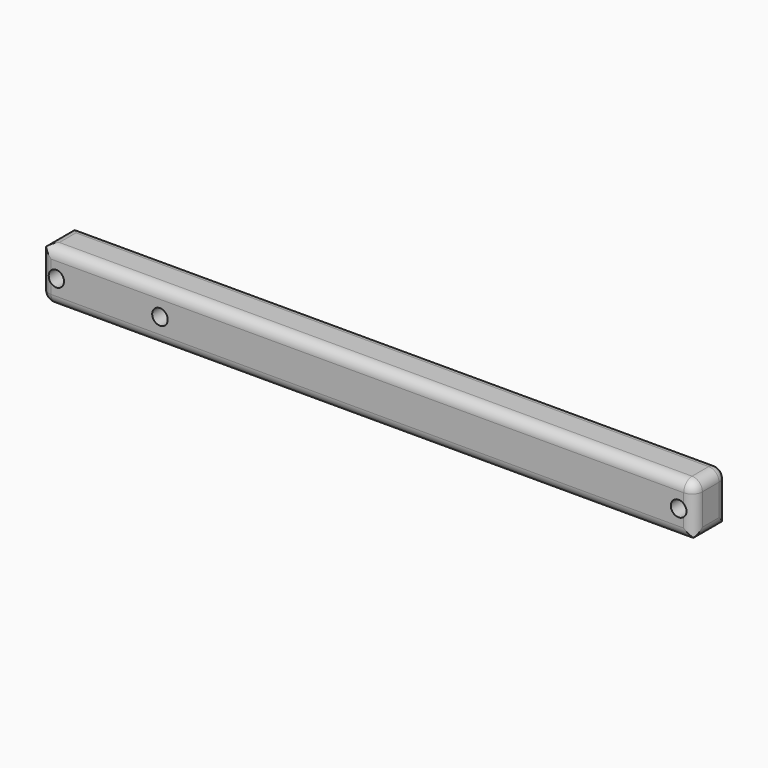
from build123d import *

# Parameters (mm, degrees)
F0_W         = 126
F0_H         = 10
F0_R         = 1.5
F1_DEPTH     = 8
F2_T1_DEPTH  = 4
F2_T3_DEPTH  = 18
F2_T5_DEPTH  = 129
F2_T7_DEPTH  = 13
F2_S11_W     = 2
F2_S11_H     = 2
F2_T12_DEPTH = 2
F2_S17_W     = 2
F2_S17_H     = 2
F2_T18_DEPTH = 2
F3_T1_DEPTH  = 11
F3_T3_DEPTH  = 4
F3_T5_DEPTH  = 127
F3_S9_W      = 2.04
F3_S9_H      = 2.04
F3_T10_DEPTH = 2.04
F3_S15_W     = 2.04
F3_S15_H     = 2.04
F3_T16_DEPTH = 2.04


# Not quite as in the source:
# - a fillet or chamfer that OpenCascade refuses, or shapes differently, is made with other operations: its cross-section is extruded or revolved along the edge and cut away or added


with BuildPart() as f1:
    # F0 (on Front) → F1 (new body)
    with BuildSketch(Plane.XZ):
        with Locations((0, 5)):
            Rectangle(F0_W, F0_H)
        with Locations((-60, 5)):
            Circle(F0_R, mode=Mode.SUBTRACT)
        with Locations((-40, 5)):
            Circle(F0_R, mode=Mode.SUBTRACT)
        with Locations((60, 5)):
            Circle(F0_R, mode=Mode.SUBTRACT)
    extrude(amount=F1_DEPTH)

    # F2: fillet of radius 2 on 7 edges, made by hand

    # F2_s2 → F2_t1 (cut)
    with BuildSketch(Plane.XZ.offset(2)):
        with BuildLine():
            ThreePointArc((63, 8), (62.4142135624, 9.4142135624), (61, 10))
            Line((61, 10), (63, 10))
            Line((63, 10), (63, 8))
        make_face()
    extrude(amount=F2_T1_DEPTH, mode=Mode.SUBTRACT)

    # F2_s4 → F2_t3 (cut)
    with BuildSketch(Plane.XZ.offset(-5)):
        with BuildLine():
            ThreePointArc((-63, 8), (-62.4142135624, 9.4142135624), (-61, 10))
            Line((-61, 10), (-63, 10))
            Line((-63, 10), (-63, 8))
        make_face()
        with BuildLine():
            ThreePointArc((61, 0), (62.4142135624, 0.5857864376), (63, 2))
            Line((63, 2), (63, 0))
            Line((63, 0), (61, 0))
        make_face()
    extrude(amount=F2_T3_DEPTH, mode=Mode.SUBTRACT)

    # F2_s6 → F2_t5 (cut)
    with BuildSketch(Plane.YZ.offset(-68)):
        with BuildLine():
            ThreePointArc((-2, 10), (-0.5857864376, 9.4142135624), (0, 8))
            Line((0, 8), (0, 10))
            Line((0, 10), (-2, 10))
        make_face()
        with BuildLine():
            ThreePointArc((-6, 10), (-7.4142135624, 9.4142135624), (-8, 8))
            Line((-8, 8), (-8, 10))
            Line((-8, 10), (-6, 10))
        make_face()
    extrude(amount=F2_T5_DEPTH, mode=Mode.SUBTRACT)

    # F2_s8 → F2_t7 (cut)
    with BuildSketch(Plane.XY.offset(-5)):
        with BuildLine():
            ThreePointArc((63, -2), (62.4142135624, -0.5857864376), (61, 0))
            Line((61, 0), (63, 0))
            Line((63, 0), (63, -2))
        make_face()
        with BuildLine():
            ThreePointArc((63, -6), (62.4142135624, -7.4142135624), (61, -8))
            Line((61, -8), (63, -8))
            Line((63, -8), (63, -6))
        make_face()
    extrude(amount=F2_T7_DEPTH, mode=Mode.SUBTRACT)


with BuildPart() as f2_tool10:
    # F2_s11 → F2_t12 (new body)
    with BuildSketch(Plane.YZ.offset(61)):
        with Locations((-1, 9)):
            Rectangle(F2_S11_W, F2_S11_H)
    extrude(amount=F2_T12_DEPTH)

    # F2_s13 → F2_t14 (revolve, cut)
    with BuildSketch(Plane(origin=(61, -2, 8), x_dir=(0, -0.7071067812, -0.7071067812), z_dir=(0, -0.7071067812, 0.7071067812))):
        with BuildLine():
            ThreePointArc((0, -2), (2, 0), (0, 2))
            Line((0, 2), (0, -2))
        make_face()
    revolve(axis=Axis((61, -2, 8), (1, 0, 0)), mode=Mode.SUBTRACT)


with BuildPart() as f1_1:
    add(f1.part)

    # F2_t9: cut F2_tool10
    add(f2_tool10.part, mode=Mode.SUBTRACT)


with BuildPart() as f2_tool16:
    # F2_s17 → F2_t18 (new body)
    with BuildSketch(Plane.XZ.offset(6)):
        with Locations((62, 9)):
            Rectangle(F2_S17_W, F2_S17_H)
    extrude(amount=F2_T18_DEPTH)

    # F2_s19 → F2_t20 (revolve, cut)
    with BuildSketch(Plane(origin=(61, -6, 8), x_dir=(-0.7071067812, 0, -0.7071067812), z_dir=(-0.7071067812, 0, 0.7071067812))):
        with BuildLine():
            ThreePointArc((0, -2), (2, 0), (0, 2))
            Line((0, 2), (0, -2))
        make_face()
    revolve(axis=Axis((61, -6, 8), (0, -1, 0)), mode=Mode.SUBTRACT)


with BuildPart() as f1_2:
    add(f1_1.part)

    # F2_t15: cut F2_tool16
    add(f2_tool16.part, mode=Mode.SUBTRACT)

    # F3: fillet of radius 2 on 7 edges, made by hand

    # F3_s2 → F3_t1 (cut)
    with BuildSketch(Plane.XY.offset(2)):
        with BuildLine():
            ThreePointArc((-63, -2), (-62.4142135624, -0.5857864376), (-61, 0))
            Line((-61, 0), (-63, 0))
            Line((-63, 0), (-63, -2))
        make_face()
        with BuildLine():
            ThreePointArc((-63, -6), (-62.4142135624, -7.4142135624), (-61, -8))
            Line((-61, -8), (-63, -8))
            Line((-63, -8), (-63, -6))
        make_face()
    extrude(amount=F3_T1_DEPTH, mode=Mode.SUBTRACT)

    # F3_s4 → F3_t3 (cut)
    with BuildSketch(Plane.XZ.offset(2)):
        with BuildLine():
            ThreePointArc((-63, 2), (-62.4142135624, 0.5857864376), (-61, 0))
            Line((-61, 0), (-63, 0))
            Line((-63, 0), (-63, 2))
        make_face()
    extrude(amount=F3_T3_DEPTH, mode=Mode.SUBTRACT)

    # F3_s6 → F3_t5 (cut)
    with BuildSketch(Plane.YZ.offset(-61)):
        with BuildLine():
            ThreePointArc((0, 2), (-0.5857864376, 0.5857864376), (-2, 0))
            Line((-2, 0), (0, 0))
            Line((0, 0), (0, 2))
        make_face()
        with BuildLine():
            ThreePointArc((-6, 0), (-7.4142135624, 0.5857864376), (-8, 2))
            Line((-8, 2), (-8, 0))
            Line((-8, 0), (-6, 0))
        make_face()
    extrude(amount=F3_T5_DEPTH, mode=Mode.SUBTRACT)


with BuildPart() as f3_tool8:
    # F3_s9 → F3_t10 (new body)
    with BuildSketch(Plane.YZ.offset(-61)):
        with Locations((-0.98, 0.98)):
            Rectangle(F3_S9_W, F3_S9_H)
    extrude(amount=-F3_T10_DEPTH)

    # F3_s11 → F3_t12 (revolve, cut)
    with BuildSketch(Plane(origin=(-61, -2, 2), x_dir=(0, -0.7071067812, 0.7071067812), z_dir=(0, -0.7071067812, -0.7071067812))):
        with BuildLine():
            ThreePointArc((0, -2), (2, 0), (0, 2))
            Line((0, 2), (0, -2))
        make_face()
    revolve(axis=Axis((-61, -2, 2), (-1, 0, 0)), mode=Mode.SUBTRACT)


with BuildPart() as f1_3:
    add(f1_2.part)

    # F3_t7: cut F3_tool8
    add(f3_tool8.part, mode=Mode.SUBTRACT)


with BuildPart() as f3_tool14:
    # F3_s15 → F3_t16 (new body)
    with BuildSketch(Plane.YZ.offset(-61)):
        with Locations((-7.02, 0.98)):
            Rectangle(F3_S15_W, F3_S15_H)
    extrude(amount=-F3_T16_DEPTH)

    # F3_s17 → F3_t18 (revolve, cut)
    with BuildSketch(Plane(origin=(-61, -6, 2), x_dir=(0, 0.7071067812, 0.7071067812), z_dir=(0, -0.7071067812, 0.7071067812))):
        with BuildLine():
            ThreePointArc((0, -2), (2, 0), (0, 2))
            Line((0, 2), (0, -2))
        make_face()
    revolve(axis=Axis((-61, -6, 2), (-1, 0, 0)), mode=Mode.SUBTRACT)


with BuildPart() as f1_4:
    add(f1_3.part)

    # F3_t13: cut F3_tool14
    add(f3_tool14.part, mode=Mode.SUBTRACT)


solid = f1_4.part
